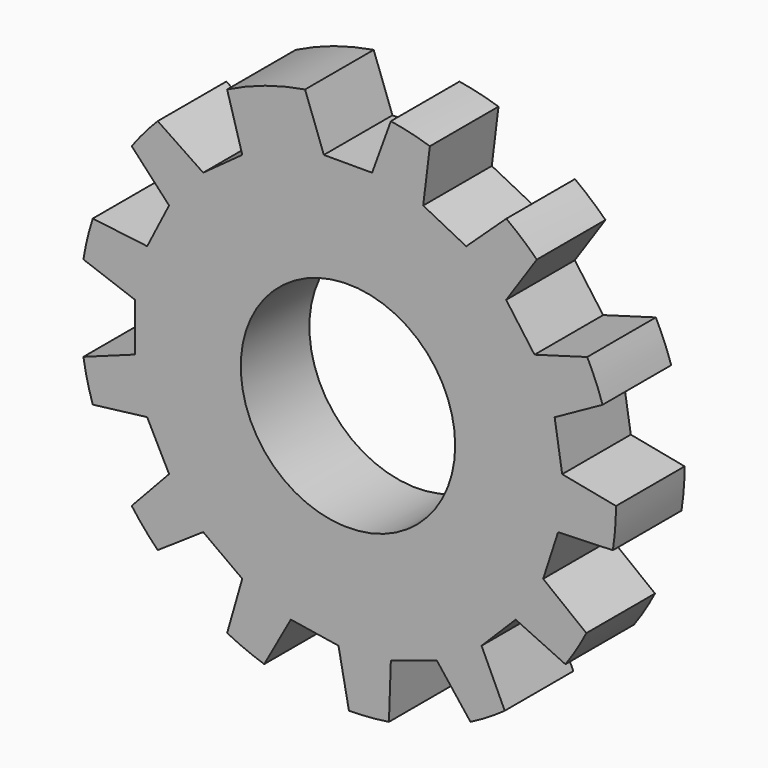
from build123d import *

# Parameters (mm, degrees)
F3_R            = 5
F4_DEPTH        = 4
F5_DEPTH        = 8
F5_COPIES_COUNT = 13
F5_COPIES_ANGLE = 324


# Not quite as in the source:
# - a feature of the source that left no trace in its solid (it failed there, or was rolled back) is left out
# - a pattern or mirror of a feature is missing from the dataset's text; its kind, count and spacing are read off the source's solid


with BuildPart() as f4:
    # F3 (on Front) → F4 (new body)
    with BuildSketch(Plane.XZ):
        with BuildLine():
            ThreePointArc((-2, 12.3389626793), (-8.100925873, -9.5197163823), (12.5, 0))
            ThreePointArc((12.5, 0), (9.5197163823, 8.100925873), (2, 12.3389626793))
            Line((2, 12.3389626793), (1.1255583585, 9.9364540145))
            Line((1.1255583585, 9.9364540145), (-1.1255583585, 9.9364540145))
            Line((-1.1255583585, 9.9364540145), (-2, 12.3389626793))
        make_face()
        Circle(F3_R, mode=Mode.SUBTRACT)
        with BuildLine():
            Line((1.1255583585, 9.9364540145), (2, 12.3389626793))
            ThreePointArc((2, 12.3389626793), (0, 12.5), (-2, 12.3389626793))
            Line((-2, 12.3389626793), (-1.1255583585, 9.9364540145))
            Line((-1.1255583585, 9.9364540145), (1.1255583585, 9.9364540145))
        make_face()
    extrude(amount=F4_DEPTH)

    # F3 (on Front) → F5 (cut)
    with BuildSketch(Plane.XZ):
        with BuildLine():
            Line((1.1255583585, 9.9364540145), (2, 12.3389626793))
            ThreePointArc((2, 12.3389626793), (0, 12.5), (-2, 12.3389626793))
            Line((-2, 12.3389626793), (-1.1255583585, 9.9364540145))
            Line((-1.1255583585, 9.9364540145), (1.1255583585, 9.9364540145))
        make_face()
    f5 = extrude(amount=F5_DEPTH, mode=Mode.SUBTRACT)

    # F5_copies: F5 ×13 about axis
    f5_copies_axis = Axis((0, 0, 0), (0, 1, 0))
    for i in range(1, F5_COPIES_COUNT):
        add(f5.rotate(f5_copies_axis, i * F5_COPIES_ANGLE / (F5_COPIES_COUNT - 1)), mode=Mode.SUBTRACT)


solid = f4.part
